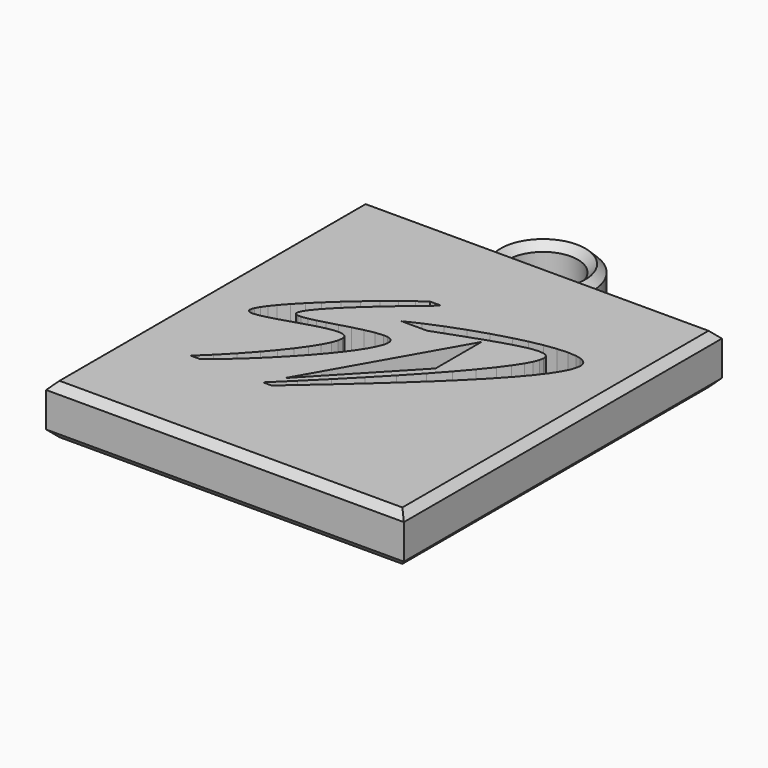
from build123d import *

# Parameters (mm, degrees)
F1_DEPTH = 10
F2_SIZE  = 1.49999
F4_DEPTH = 10


# Not quite as in the source:
# - a fillet or chamfer is up to 0.001 mm smaller than in the source, because OpenCascade refuses the exact size


with BuildPart() as f1:
    # F0 (on Top) → F1 (new body)
    with BuildSketch(Plane.XY):
        with BuildLine():
            Line((7.0000007749, 40), (10, 40))
            ThreePointArc((10, 40), (0, 50), (-10, 40))
            Line((-10, 40), (-7.0000007749, 40))
            ThreePointArc((-7.0000007749, 40), (0, 47.0000007749), (7.0000007749, 40))
        make_face()
        Polygon((36, -40), (36, 40), (10, 40), (7.0000007749, 40), (-7.0000007749, 40), (-10, 40), (-36, 40), (-36, -40), align=None)
    extrude(amount=F1_DEPTH)

    # F2 (size 1.5 in the source; OpenCascade refuses exactly that, so slightly less here)
    f2_edges = [f1.edges().sort_by_distance(p)[0] for p in [
        (0, 50, 10),
        (-23, 40, 10),
        (-36, 0, 10),
        (0, -40, 10),
        (36, 0, 10),
        (23, 40, 10),
        (0, 47.000001, 10),
        (0, 40, 10),
        (0, 50, 0),
        (-23, 40, 0),
        (-36, 0, 0),
        (0, -40, 0),
        (36, 0, 0),
        (23, 40, 0),
        (0, 47.000001, 0),
        (0, 40, 0),
    ]]
    chamfer(f2_edges, length=F2_SIZE)

    # F3 (on face) → F4 (cut)
    with BuildSketch(Plane.XY.offset(10)):
        Polygon((9.01941, 13.251642), (-7.413878, -15.645048), (9.01941, 1.689704), align=None)
        Polygon((-5.229314, 10.897392), (-0.043674, 10.897392), (2.962569, 11.978135), (5.871741, 13.023694), (8.637504, 13.995209), (11.213521, 14.853819), (13.553455, 15.560666), (15.610967, 16.076888), (16.940888, 16.315581), (18.066333, 16.408794), (18.967754, 16.340134), (19.485045, 16.172547), (19.857078, 15.897769), (20.075875, 15.509104), (20.140122, 15.005391), (19.980223, 14.112285), (19.543063, 13.014817), (18.845257, 11.726576), (17.710823, 9.98186), (16.264623, 8.013275), (14.174175, 5.408678), (11.72632, 2.555867), (8.966951, -0.507624), (5.716937, -3.981084), (2.218444, -7.607146), (-1.472083, -11.339644), (-5.298199, -15.132416), (-9.20346, -18.939297), (-7.467058, -18.939297), (-3.873072, -15.801826), (-0.094887, -12.481081), (3.769463, -9.040146), (7.621943, -5.542107), (11.36452, -2.050048), (14.671952, 1.148161), (17.718542, 4.234917), (20.424586, 7.15893), (22.376178, 9.451811), (23.983998, 11.56327), (25.043446, 13.189903), (25.792536, 14.645471), (26.202411, 15.911404), (26.271608, 16.686717), (26.143923, 17.349851), (25.809161, 17.894215), (25.267338, 18.318258), (24.53297, 18.627591), (23.621676, 18.82837), (21.854292, 18.939297), (19.744262, 18.817766), (17.353663, 18.488244), (14.744575, 17.975197), (11.979075, 17.30309), (8.331078, 16.256236), (4.658259, 15.041801), (1.0886, 13.710223), (-2.249918, 12.31194), align=None)
        Polygon((-5.840144, 17.088177), (-3.619251, 18.933561), (-5.855152, 18.933561), (-7.766318, 17.582905), (-9.890915, 15.963704), (-12.153333, 14.1388), (-14.477963, 12.171034), (-16.789194, 10.123247), (-19.011419, 8.058281), (-20.833308, 6.276802), (-22.476192, 4.573508), (-23.888546, 2.991223), (-24.802964, 1.860788), (-25.518263, 0.852267), (-26.00945, -0.013567), (-26.195816, -0.487065), (-26.271609, -0.886829), (-26.230101, -1.207268), (-26.064565, -1.442791), (-25.726944, -1.601419), (-25.239428, -1.656759), (-24.209316, -1.56342), (-22.607846, -1.213122), (-20.724778, -0.679711), (-18.671706, -0.044733), (-16.560227, 0.610268), (-14.501933, 1.203748), (-13.152533, 1.53891), (-11.922154, 1.776), (-10.849071, 1.887047), (-9.838371, 1.818066), (-9.158572, 1.492121), (-8.872137, 1.070319), (-8.770299, 0.510027), (-8.901347, -0.43259), (-9.311798, -1.573728), (-10.129528, -3.159215), (-11.258734, -4.942681), (-12.651899, -6.877665), (-14.261505, -8.917703), (-16.040031, -11.016334), (-18.545222, -13.775636), (-21.151889, -16.451403), (-23.753323, -18.939297), (-21.841571, -18.939297), (-19.26416, -16.826499), (-16.566892, -14.424306), (-13.846275, -11.824217), (-11.198816, -9.11773), (-9.327369, -7.082132), (-7.590687, -5.076318), (-6.028942, -3.138376), (-4.738285, -1.386829), (-3.678568, 0.235044), (-2.884733, 1.694116), (-2.391719, 2.957258), (-2.24357, 3.715625), (-2.276453, 4.347186), (-2.5028, 4.840154), (-2.934991, 5.182783), (-3.574073, 5.372), (-4.395773, 5.424114), (-6.021186, 5.269587), (-7.929695, 4.890115), (-10.007823, 4.363257), (-12.142089, 3.766577), (-14.219015, 3.177635), (-15.808866, 2.752566), (-17.218733, 2.429106), (-18.505432, 2.241234), (-19.124111, 2.244482), (-19.559671, 2.362015), (-19.803219, 2.624939), (-19.830168, 3.023301), (-19.558342, 3.744641), (-18.971466, 4.657578), (-17.935128, 5.935143), (-16.584765, 7.39239), (-14.985004, 8.983921), (-13.200474, 10.664336), (-10.763992, 12.85997), (-8.266136, 15.032448), align=None)
    extrude(amount=-F4_DEPTH, mode=Mode.SUBTRACT)


solid = f1.part
